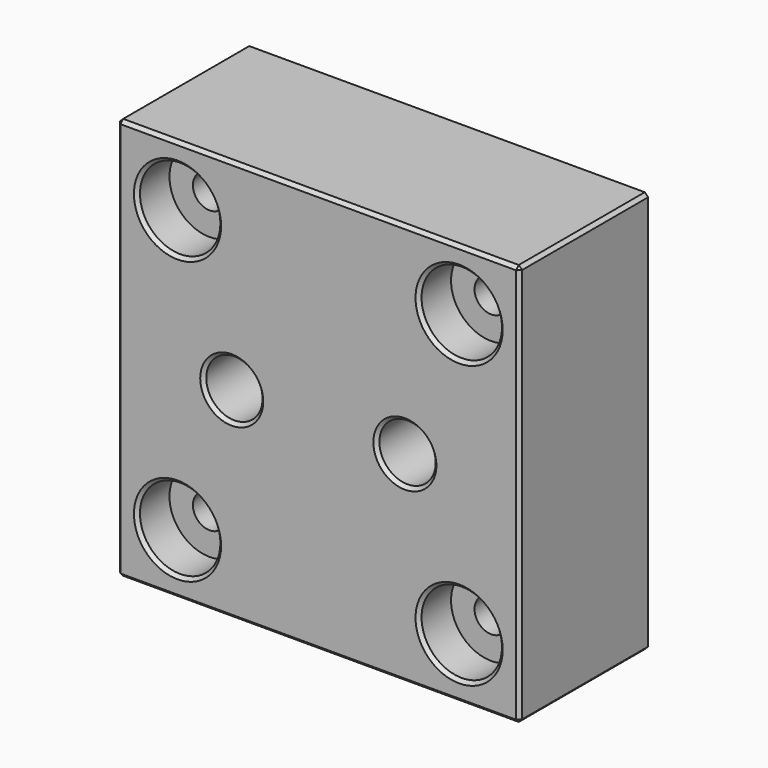
from build123d import *

# Parameters (mm, degrees)
F0_W      = 30
F0_H      = 30
F0_R      = 10
F0_R_2    = 3
F1_DEPTH  = 12
F2_R      = 1.25
F3_DEPTH  = 20
F4_DEPTH  = 3
F5_R      = 3
F5_R_2    = 1.25
F6_DEPTH  = 3
F8_DEPTH  = 3
F9_DEPTH  = 3
F12_D     = 3
F14_D     = 4.2
F14_DEPTH = 5
F14_TIP   = 1.2618073
F15_SIZE  = 0.25


# Not quite as in the source:
# - a feature names something its author has since deleted; it is built from what else it names


with BuildPart() as f1:
    # F0 (on Front) → F1 (new body)
    with BuildSketch(Plane.XZ):
        with Locations((15, -15)):
            Rectangle(F0_W, F0_H)
        with Locations((15, -15)):
            Circle(F0_R, mode=Mode.SUBTRACT)
        with Locations((15, -15)):
            Circle(F0_R)
        with Locations((15, -16.066)):
            Circle(F0_R_2, mode=Mode.SUBTRACT)
        with Locations((15, -16.066)):
            Circle(F0_R_2)
    extrude(amount=F1_DEPTH)

    # F2 (on face) → F3 (cut)
    with BuildSketch(Plane(origin=(0, 0, 0), x_dir=(-1, 0, 0), z_dir=(0, 1, 0))):
        with Locations((-4.5, -4.5)):
            Circle(F2_R)
        with Locations((-25.5, -4.5)):
            Circle(F2_R)
        with Locations((-25.5, -25.5)):
            Circle(F2_R)
        with Locations((-4.5, -25.5)):
            Circle(F2_R)
    extrude(amount=-F3_DEPTH, mode=Mode.SUBTRACT)

    # F0 (on Front) → F4 (cut)
    with BuildSketch(Plane.XZ):
        with Locations((15, -16.066)):
            Circle(F0_R_2)
    extrude(amount=F4_DEPTH, mode=Mode.SUBTRACT)

    # F5 (on face) → F6 (cut)
    with BuildSketch(Plane.XZ.offset(12)):
        with Locations((4.5, -4.5)):
            Circle(F5_R)
        with Locations((4.5, -4.5)):
            Circle(F5_R_2, mode=Mode.SUBTRACT)
        with Locations((25.5, -4.5)):
            Circle(F5_R)
        with Locations((25.5, -4.5)):
            Circle(F5_R_2, mode=Mode.SUBTRACT)
        with Locations((4.5, -25.5)):
            Circle(F5_R)
        with Locations((4.5, -25.5)):
            Circle(F5_R_2, mode=Mode.SUBTRACT)
        with Locations((25.5, -25.5)):
            Circle(F5_R)
        with Locations((25.5, -25.5)):
            Circle(F5_R_2, mode=Mode.SUBTRACT)
    extrude(amount=-F6_DEPTH, mode=Mode.SUBTRACT)

    # F7 (on face) → F8 (cut)
    with BuildSketch(Plane(origin=(0, 0, 0), x_dir=(-1, 0, 0), z_dir=(0, 1, 0))):
        with BuildLine():
            Line((-17.9580398915, -15.566), (-19.9749371855, -15.566))
            ThreePointArc((-19.9749371855, -15.566), (-20, -16.066), (-19.9749371855, -16.566))
            Line((-19.9749371855, -16.566), (-17.9580398915, -16.566))
            ThreePointArc((-17.9580398915, -16.566), (-18, -16.066), (-17.9580398915, -15.566))
        make_face()
    extrude(amount=-F8_DEPTH, mode=Mode.SUBTRACT)

    # F7 (on face) → F9 (cut)
    with BuildSketch(Plane(origin=(0, 0, 0), x_dir=(-1, 0, 0), z_dir=(0, 1, 0))):
        with BuildLine():
            ThreePointArc((-18.4208497185, -12.4193868859), (-18.4150519192, -9.7016030586), (-21.128355545, -9.8576991225))
            ThreePointArc((-21.128355545, -9.8576991225), (-22.8195543866, -16.6895470386), (-18.4586259046, -22.2137304394))
            ThreePointArc((-18.4586259046, -22.2137304394), (-17.1046358453, -21.7662439553), (-17.5, -20.3961270189))
            ThreePointArc((-17.5, -20.3961270189), (-19.1995404186, -18.7796433577), (-19.9749371855, -16.566))
            Line((-19.9749371855, -16.566), (-21.5030275285, -16.566))
            ThreePointArc((-21.5030275285, -16.566), (-22.0030275285, -16.066), (-21.5030275285, -15.566))
            Line((-21.5030275285, -15.566), (-19.9749371855, -15.566))
            ThreePointArc((-19.9749371855, -15.566), (-19.4830350162, -13.8518642672), (-18.4208497185, -12.4193868859))
        make_face()
        with BuildLine():
            ThreePointArc((-11.5413740954, -22.2137304394), (-7.1804456134, -16.6895470386), (-8.871644455, -9.8576991225))
            ThreePointArc((-8.871644455, -9.8576991225), (-11.5849480808, -9.7016030586), (-11.5791502815, -12.4193868859))
            ThreePointArc((-11.5791502815, -12.4193868859), (-10.0329877054, -16.6394011384), (-12.5, -20.3961270189))
            ThreePointArc((-12.5, -20.3961270189), (-12.8953641547, -21.7662439553), (-11.5413740954, -22.2137304394))
        make_face()
        with BuildLine():
            ThreePointArc((-19.9749371855, -16.566), (-20, -16.066), (-19.9749371855, -15.566))
            Line((-19.9749371855, -15.566), (-21.5030275285, -15.566))
            ThreePointArc((-21.5030275285, -15.566), (-22.0030275285, -16.066), (-21.5030275285, -16.566))
            Line((-21.5030275285, -16.566), (-19.9749371855, -16.566))
        make_face()
    extrude(amount=-F9_DEPTH, mode=Mode.SUBTRACT)

    # F12 (through all)
    with Locations(Plane(origin=(0, 0, 0), x_dir=(-1, 0, 0), z_dir=(0, 1, 0))):
        with Locations((-21.456294, -15), (-8.543706, -15)):
            Hole(F12_D / 2)

    # F14
    with Locations(Plane.XZ.offset(12)):
        with Locations((8.543706, -15), (21.456294, -15)):
            Hole(F14_D / 2, depth=F14_DEPTH)
            with Locations((0, 0, -(F14_DEPTH + F14_TIP / 2))):  # 118° drill point
                Cone(0, F14_D / 2, F14_TIP, mode=Mode.SUBTRACT)

    # F15
    f15_edges = [f1.edges().sort_by_distance(p)[0] for p in [
        (15, -12, 0),
        (30, -12, -15),
        (0, -12, -15),
        (15, -12, -30),
        (1.5, -12, -25.5),
        (22.5, -12, -25.5),
        (6.443706, -12, -15),
        (1.5, -12, -4.5),
        (19.356294, -12, -15),
        (22.5, -12, -4.5),
        (0, -6, 0),
        (30, -6, 0),
        (30, -6, -30),
        (0, -6, -30),
    ]]
    chamfer(f15_edges, length=F15_SIZE)


solid = f1.part
